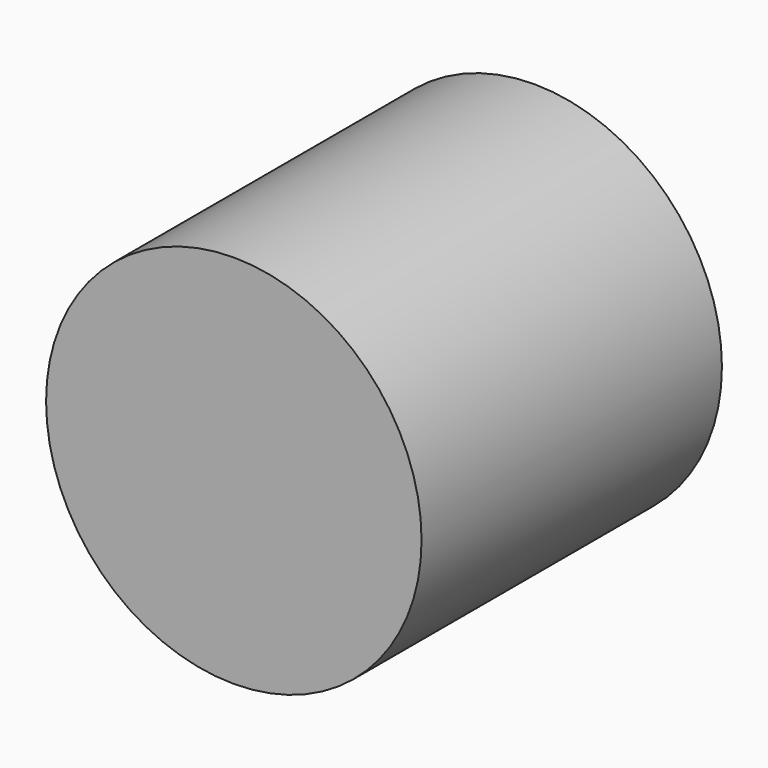
from build123d import *

# Parameters (mm, degrees)
F0_R     = 25.4
F1_DEPTH = 25.4


# Not quite as in the source:
# - the program builds the solid bodies; features that only make, move or delete a surface that nothing else refers to are left out


with BuildPart() as f1:
    # F0 (on Front) → F1 (new body, symmetric)
    with BuildSketch(Plane.XZ):
        Circle(F0_R)
    extrude(amount=F1_DEPTH, both=True)


solid = f1.part
